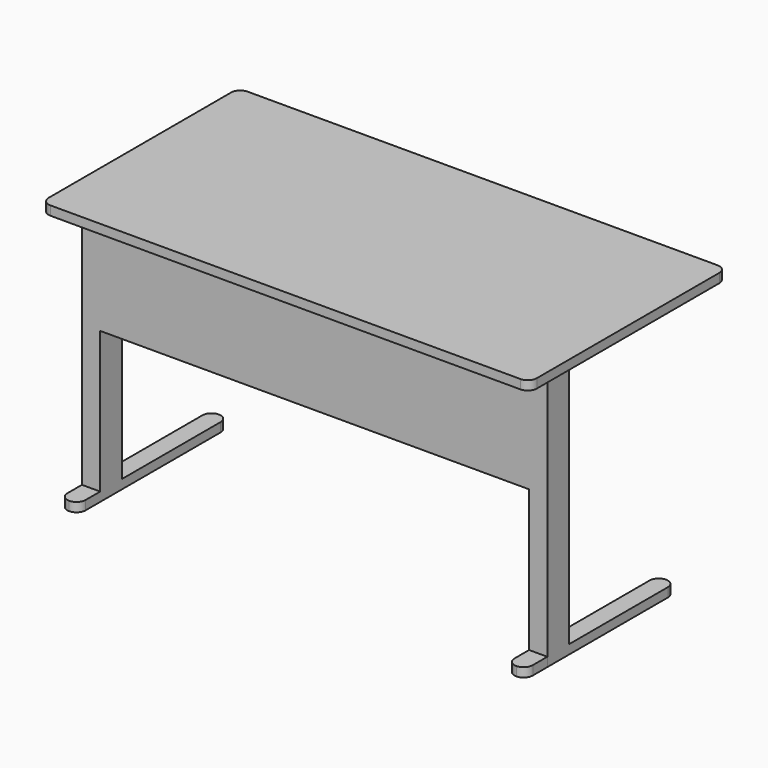
from build123d import *

# Parameters (mm, degrees)
F1_DEPTH  = 25.4
F2_W      = 50.8
F2_H      = 25.4
F3_DEPTH  = 25.4
F5_DEPTH  = 673.1
F4_W      = 1193.8120010341
F4_H      = 25.4
F7_DEPTH  = 25.4
F8_DEPTH  = 279.4
F9_W      = 50.728738308
F9_H      = 76.2
F10_DEPTH = 25.4
F11_W     = 50.8
F11_H     = 76.2
F12_DEPTH = 25.4


# Not quite as in the source:
# - ends of sketch curves that miss each other by under 0.0002 mm in the source are joined


with BuildPart() as f1:
    # F0 (on Top) → F1 (new body)
    with BuildSketch(Plane.XY):
        with BuildLine():
            Line((715.1671976125, 685.8), (-592.9328023875, 685.8))
            ThreePointArc((-592.9328023875, 685.8), (-610.8933146297, 678.3605122421), (-618.3328023875, 660.4))
            Line((-618.3328023875, 660.4), (-618.3328023875, 25.4))
            ThreePointArc((-618.3328023875, 25.4), (-610.8933146297, 7.4394877579), (-592.9328023875, 0))
            Line((-592.9328023875, 0), (715.1671976125, 0))
            ThreePointArc((715.1671976125, 0), (733.1277098546, 7.4394877579), (740.5671976125, 25.4))
            Line((740.5671976125, 25.4), (740.5671976125, 660.4))
            ThreePointArc((740.5671976125, 660.4), (733.1277098546, 678.3605122421), (715.1671976125, 685.8))
        make_face()
    extrude(amount=F1_DEPTH)

    # F2 (on face) → F3 (join)
    with BuildSketch(Plane(origin=(0, 0, 0), x_dir=(1, 0, 0), z_dir=(0, 0, -1))):
        with Locations((-561.1828023875, -114.3)):
            Rectangle(F2_W, F2_H)
        with BuildLine():
            Line((-535.7828023875, -127), (-586.5828023875, -127))
            Line((-586.5828023875, -127), (-586.5828023875, -533.4))
            ThreePointArc((-586.5828023875, -533.4), (-579.1433146297, -551.3605122421), (-561.1828023875, -558.8))
            ThreePointArc((-561.1828023875, -558.8), (-543.2222901454, -551.3605122421), (-535.7828023875, -533.4))
            Line((-535.7828023875, -533.4), (-535.7828023875, -127))
        make_face()
        with BuildLine():
            Line((708.8171976125, -127), (658.0171976125, -127))
            Line((658.0171976125, -127), (658.0171976125, -533.4))
            ThreePointArc((658.0171976125, -533.4), (665.4566853703, -551.3605122421), (683.4171976125, -558.8))
            ThreePointArc((683.4171976125, -558.8), (701.3777098546, -551.3605122421), (708.8171976125, -533.4))
            Line((708.8171976125, -533.4), (708.8171976125, -127))
        make_face()
        with Locations((683.4171976125, -114.3)):
            Rectangle(F2_W, F2_H)
    extrude(amount=F3_DEPTH)

    # F4 (on face) → F5 (join)
    with BuildSketch(Plane(origin=(0, 0, -25.4), x_dir=(1, 0, 0), z_dir=(0, 0, -1))):
        Polygon((-535.7828023875, -127), (-535.7828023875, -101.6), (-586.5828023875, -101.6), (-586.5828023875, -177.8), (-535.7828023875, -177.8), align=None)
        Polygon((708.7579369545, -101.6), (658.0291986465, -101.6), (658.0291986465, -127), (658.0291986465, -177.8), (708.7579369545, -177.8), align=None)
    extrude(amount=F5_DEPTH)

    # F4 (on face) → F7 (join)
    with BuildSketch(Plane(origin=(0, 0, -25.4), x_dir=(1, 0, 0), z_dir=(0, 0, -1))):
        with Locations((61.1231981295, -114.3)):
            Rectangle(F4_W, F4_H)
    extrude(amount=-F7_DEPTH)

    # F4 (on face) → F8 (join)
    with BuildSketch(Plane(origin=(0, 0, -25.4), x_dir=(1, 0, 0), z_dir=(0, 0, -1))):
        with Locations((61.1231981295, -114.3)):
            Rectangle(F4_W, F4_H)
    extrude(amount=F8_DEPTH)

    # F9 (on face) → F10 (join)
    with BuildSketch(Plane(origin=(0, 0, -698.5), x_dir=(1, 0, 0), z_dir=(0, 0, -1))):
        with BuildLine():
            Line((708.7579369545, -177.8), (658.0291986465, -177.8))
            Line((658.0291986465, -177.8), (658.0291986465, -520.7))
            ThreePointArc((658.0291986465, -520.7), (665.4435093373, -538.6352998323), (683.357937235, -546.0999000355))
            Line((683.357937235, -546.0999000355), (683.4291986465, -546.1))
            ThreePointArc((683.4291986465, -546.1), (701.3436262637, -538.6352998323), (708.7579369545, -520.7))
            Line((708.7579369545, -520.7), (708.7579369545, -177.8))
        make_face()
        with Locations((683.3935678005, -139.7)):
            Rectangle(F9_W, F9_H)
        with BuildLine():
            Line((658.0291986465, -50.8), (658.0291986465, -101.6))
            Line((658.0291986465, -101.6), (708.7579369545, -101.6))
            Line((708.7579369545, -101.6), (708.8171976125, -101.6))
            Line((708.8171976125, -101.6), (708.8171976125, -50.8))
            ThreePointArc((708.8171976125, -50.8), (701.3819523594, -32.843731265), (683.4291986452, -25.4000028351))
            Line((683.4291986452, -25.4000028351), (683.4171976125, -25.4))
            ThreePointArc((683.4171976125, -25.4), (665.4644438997, -32.843731265), (658.0291986465, -50.8))
        make_face()
    extrude(amount=F10_DEPTH)

    # F11 (on face) → F12 (join)
    with BuildSketch(Plane(origin=(0, 0, -698.5), x_dir=(1, 0, 0), z_dir=(0, 0, -1))):
        with BuildLine():
            ThreePointArc((-561.1828023875, -25.4), (-579.1433146297, -32.8394877579), (-586.5828023875, -50.8))
            Line((-586.5828023875, -50.8), (-586.5828023875, -101.6))
            Line((-586.5828023875, -101.6), (-535.7828023875, -101.6))
            Line((-535.7828023875, -101.6), (-535.7828023875, -50.8))
            ThreePointArc((-535.7828023875, -50.8), (-543.2222901454, -32.8394877579), (-561.1828023875, -25.4))
        make_face()
        with Locations((-561.1828023875, -139.7)):
            Rectangle(F11_W, F11_H)
        with BuildLine():
            Line((-535.7828023875, -177.8), (-586.5828023875, -177.8))
            Line((-586.5828023875, -177.8), (-586.5828023875, -520.7))
            ThreePointArc((-586.5828023875, -520.7), (-579.1433146297, -538.6605122421), (-561.1828023875, -546.1))
            ThreePointArc((-561.1828023875, -546.1), (-543.2222901454, -538.6605122421), (-535.7828023875, -520.7))
            Line((-535.7828023875, -520.7), (-535.7828023875, -177.8))
        make_face()
    extrude(amount=F12_DEPTH)


solid = f1.part
